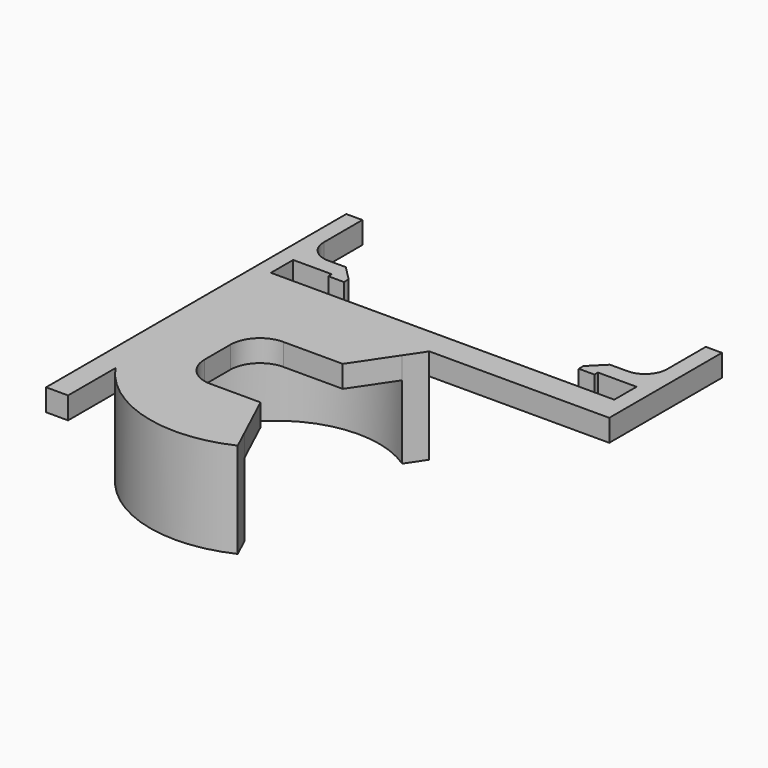
from build123d import *

# Parameters (mm, degrees)
F0_W     = 1.1
F0_H     = 4.7914452539
F1_DEPTH = 1.5
F2_SIZE  = 1
F3_R     = 1.5
F5_DEPTH = 1.5
F6_DEPTH = 5
F7_R     = 2


# Not quite as in the source:
# - a feature names something its author has since deleted; it is built from what else it names


with BuildPart() as f1:
    # F0 (on Top) → F1 (new body)
    with BuildSketch(Plane.XY):
        with BuildLine():
            ThreePointArc((-8.55, 0), (-4.0253321977, 7.5431558845), (4.7597545494, 7.1026218138))
            Line((4.7597545494, 7.1026218138), (4.7907789053, 7.1026218138))
            Line((4.7907789053, 7.1026218138), (6.0061305772, 8.9044547655))
            Line((6.0061305772, 8.9044547655), (-7.45, 8.9044547655))
            Line((-7.45, 8.9044547655), (-7.45, 10.8044547655))
            Line((-7.45, 10.8044547655), (-4.820069465, 10.8044547655))
            Line((-4.820069465, 10.8044547655), (-4.820069465, 10.5132658899))
            Line((-4.820069465, 10.5132658899), (-3.75, 10.5044547655))
            Line((-3.75, 10.5044547655), (-3.75, 10.8044547655))
            Line((-3.75, 10.8044547655), (-3.75, 11.9085547461))
            Line((-3.75, 11.9085547461), (-7.45, 11.9085547461))
            Line((-7.45, 11.9085547461), (-8.55, 11.9085547461))
            Line((-8.55, 11.9085547461), (-8.55, 10.5085547461))
            Line((-8.55, 10.5085547461), (-8.55, 0))
        make_face()
        with BuildLine():
            Line((-7.05, -8.869094649), (-7.05, -4.837354649))
            ThreePointArc((-7.05, -4.837354649), (-8.1663945533, -2.5322914524), (-8.55, 0))
            Line((-8.55, 0), (-8.55, -8.869094649))
            Line((-8.55, -8.869094649), (-7.05, -8.869094649))
        make_face()
        with BuildLine():
            ThreePointArc((2.9794587453, -6.3894698986), (-7.0282672028, 0.5531366249), (3.9423099695, 5.8447148865))
            Line((3.9423099695, 5.8447148865), (4.7810993247, 7.0882712453))
            ThreePointArc((4.7810993247, 7.0882712453), (4.7704323333, 7.0954545558), (4.7597545494, 7.1026218138))
            ThreePointArc((4.7597545494, 7.1026218138), (-4.0253321977, 7.5431558845), (-8.55, 0))
            ThreePointArc((-8.55, 0), (-8.1663945533, -2.5322914524), (-7.05, -4.837354649))
            ThreePointArc((-7.05, -4.837354649), (-2.2520876458, -8.248066515), (3.6133861379, -7.7489315792))
            Line((3.6133861379, -7.7489315792), (2.9794587453, -6.3894698986))
        make_face()
        Polygon((6.0061305772, 8.9044547655), (4.7907789053, 7.1026218138), (15.4494866027, 7.1026218138), (17.05, 7.1026218138), (17.05, 11.9085547461), (15.95, 11.9085547461), (12.25, 11.9085547461), (12.25, 10.8044547655), (12.25, 10.5044547655), (13.32, 10.5044547655), (13.32, 10.8044547655), (15.95, 10.8044547655), (15.95, 8.9044547655), align=None)
        with Locations((-8, 14.3042773731)):
            Rectangle(F0_W, F0_H)
        with Locations((16.5, 14.3042773731)):
            Rectangle(F0_W, F0_H)
    extrude(amount=F1_DEPTH)

    # F2
    f2_edges = [f1.edges().sort_by_distance(p)[0] for p in [
        (-3.75, 11.908555, 0.75),
        (12.25, 11.908555, 0.75),
    ]]
    chamfer(f2_edges, length=F2_SIZE)

    # F3
    f3_edges = [f1.edges().sort_by_distance(p)[0] for p in [
        (-7.45, 11.908555, 0.75),
        (15.95, 11.908555, 0.75),
    ]]
    fillet(f3_edges, radius=F3_R)

    # F4 (on face) → F5 (join)
    with BuildSketch(Plane.XY.offset(1.5)):
        with BuildLine():
            Line((2.0909764022, 3.1), (3.9423099695, 5.8447148865))
            ThreePointArc((3.9423099695, 5.8447148865), (-7.0282672028, 0.5531366249), (2.9794587453, -6.3894698986))
            Line((2.9794587453, -6.3894698986), (1.4455537403, -3.1))
            Line((1.4455537403, -3.1), (-3.96, -3.1))
            Line((-3.96, -3.1), (-3.96, 3.1))
            Line((-3.96, 3.1), (2.0909764022, 3.1))
        make_face()
    extrude(amount=-F5_DEPTH)

    # F0 (on Top) → F6 (join)
    with BuildSketch(Plane.XY):
        with BuildLine():
            ThreePointArc((2.9794587453, -6.3894698986), (-7.0282672028, 0.5531366249), (3.9423099695, 5.8447148865))
            Line((3.9423099695, 5.8447148865), (4.7810993247, 7.0882712453))
            ThreePointArc((4.7810993247, 7.0882712453), (4.7704323333, 7.0954545558), (4.7597545494, 7.1026218138))
            ThreePointArc((4.7597545494, 7.1026218138), (-4.0253321977, 7.5431558845), (-8.55, 0))
            ThreePointArc((-8.55, 0), (-8.1663945533, -2.5322914524), (-7.05, -4.837354649))
            ThreePointArc((-7.05, -4.837354649), (-2.2520876458, -8.248066515), (3.6133861379, -7.7489315792))
            Line((3.6133861379, -7.7489315792), (2.9794587453, -6.3894698986))
        make_face()
    extrude(amount=-F6_DEPTH)

    # F7
    f7_edges = [f1.edges().sort_by_distance(p)[0] for p in [
        (-3.96, 3.1, 0.75),
        (-3.96, -3.1, 0.75),
    ]]
    fillet(f7_edges, radius=F7_R)


solid = f1.part
